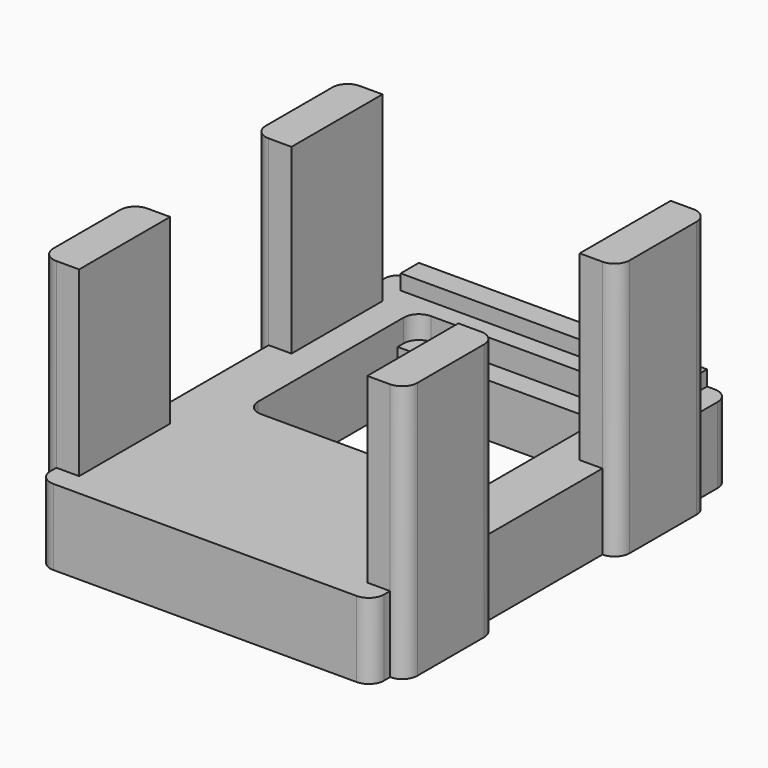
from build123d import *

# Parameters (mm, degrees)
F0_W     = 44
F0_H     = 59
F0_W_2   = 30
F0_H_2   = 22
F1_DEPTH = 10
F2_W     = 30
F2_H     = 3
F3_DEPTH = 3
F4_W     = 38
F4_H     = 3
F5_DEPTH = 2
F6_W     = 3
F6_H     = 15
F6_W_2   = 2
F7_DEPTH = 24
F8_DEPTH = 10
F9_R     = 1.99999


# Not quite as in the source:
# - a fillet or chamfer is up to 0.001 mm smaller than in the source, because OpenCascade refuses the exact size


with BuildPart() as f1:
    # F0 (on Top) → F1 (new body)
    with BuildSketch(Plane.XY):
        with Locations((0, -11)):
            Rectangle(F0_W, F0_H)
        with Locations((0, -1)):
            Rectangle(F0_W_2, F0_H_2, mode=Mode.SUBTRACT)
    extrude(amount=F1_DEPTH)

    # F2 (on face) → F3 (cut)
    with BuildSketch(Plane.XY.offset(10)):
        with Locations((0, -13.5)):
            Rectangle(F2_W, F2_H)
        with Locations((0, 11.5)):
            Rectangle(F2_W, F2_H)
    extrude(amount=-F3_DEPTH, mode=Mode.SUBTRACT)

    # F4 (on face) → F5 (join)
    with BuildSketch(Plane.XY.offset(10)):
        with Locations((0, 17)):
            Rectangle(F4_W, F4_H)
    extrude(amount=F5_DEPTH)

    # F6 (on face) → F7 (join)
    with BuildSketch(Plane.XY.offset(10)):
        with Locations((-20.5, 5)):
            Rectangle(F6_W, F6_H)
        with Locations((-23, 5)):
            Rectangle(F6_W_2, F6_H)
        with Locations((-23, -30)):
            Rectangle(F6_W_2, F6_H)
        with Locations((-20.5, -30)):
            Rectangle(F6_W, F6_H)
        with Locations((23, 5)):
            Rectangle(F6_W_2, F6_H)
        with Locations((23, -30)):
            Rectangle(F6_W_2, F6_H)
        with Locations((20.5, -30)):
            Rectangle(F6_W, F6_H)
        with Locations((20.5, 5)):
            Rectangle(F6_W, F6_H)
    extrude(amount=F7_DEPTH)

    # F6 (on face) → F8 (join, through all)
    with BuildSketch(Plane.XY.offset(10)):
        with Locations((-23, -30)):
            Rectangle(F6_W_2, F6_H)
        with Locations((-23, 5)):
            Rectangle(F6_W_2, F6_H)
        with Locations((23, -30)):
            Rectangle(F6_W_2, F6_H)
        with Locations((23, 5)):
            Rectangle(F6_W_2, F6_H)
    extrude(amount=-F8_DEPTH)

    # F9 (radius 2 in the source; OpenCascade refuses exactly that, so slightly less here)
    f9_edges = [f1.edges().sort_by_distance(p)[0] for p in [
        (24, 12.5, 17),
        (-24, 12.5, 17),
        (-24, -2.5, 17),
        (-24, -22.5, 17),
        (-24, -37.5, 17),
        (24, -37.5, 17),
        (24, -22.5, 17),
        (22, -40.5, 5),
        (-22, -40.5, 5),
        (22, 18.5, 5),
        (-22, 18.5, 5),
        (24, -2.5, 17),
        (-15, 13, 8.5),
        (15, 13, 8.5),
        (-15, -15, 8.5),
        (15, -15, 8.5),
    ]]
    fillet(f9_edges, radius=F9_R)


solid = f1.part
